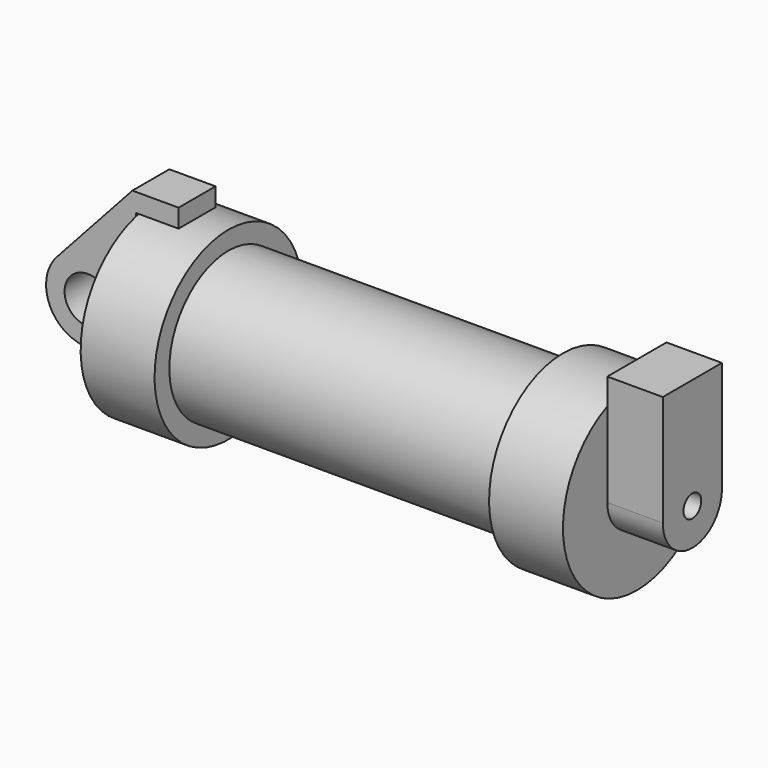
from build123d import *

# Parameters (mm, degrees)
F0_W     = 5.842
F0_H     = 12.7
F0_R     = 3.175
F2_DEPTH = 3.175
F3_R     = 1.524
F4_DEPTH = 7.62


# Not quite as in the source:
# - the program builds the solid bodies; features that only make, move or delete a surface that nothing else refers to are left out


with BuildPart() as f1:
    # F0 (on Front) → F1 (revolve)
    with BuildSketch(Plane.XZ):
        Polygon((5.842, 12.7), (5.842, 0), (66.294, 0), (66.294, 12.7), (56.134, 12.7), (56.134, 10.16), (10.16, 10.16), (10.16, 12.7), align=None)
        with Locations((2.921, 6.35)):
            Rectangle(F0_W, F0_H)
    revolve(axis=Axis((33.147, 0, 0), (-1, 0, 0)))

    # F3 (on face) → F4 (join)
    with BuildSketch(Plane.YZ.offset(66.294)):
        with BuildLine():
            ThreePointArc((-5.08, 0), (0, 5.08), (5.08, 0))
            Line((5.08, 0), (5.08, 11.6397422652))
            ThreePointArc((5.08, 11.6397422652), (0, 12.7), (-5.08, 11.6397422652))
            Line((-5.08, 11.6397422652), (-5.08, 0))
        make_face()
        with BuildLine():
            ThreePointArc((-5.08, 11.6397422652), (0, 12.7), (5.08, 11.6397422652))
            Line((5.08, 11.6397422652), (5.08, 15.24))
            Line((5.08, 15.24), (-5.08, 15.24))
            Line((-5.08, 15.24), (-5.08, 11.6397422652))
        make_face()
        with BuildLine():
            ThreePointArc((-5.08, 0), (0, -5.08), (5.08, 0))
            ThreePointArc((5.08, 0), (0, 5.08), (-5.08, 0))
        make_face()
        Circle(F3_R, mode=Mode.SUBTRACT)
    extrude(amount=F4_DEPTH)


with BuildPart() as f2:
    # F0 (on Front) → F2 (new body, symmetric)
    with BuildSketch(Plane.XZ):
        with BuildLine():
            ThreePointArc((-8.1826630726, -5.5069827884), (-3.1957909266, -4.5493385486), (-0.9398, 0))
            ThreePointArc((-0.9398, 0), (-4.5919612295, 5.3297205562), (-10.8806298187, 3.8475430269))
            ThreePointArc((-10.8806298187, 3.8475430269), (-12.1459778134, -1.5837270034), (-8.1826630726, -5.5069827884))
        make_face()
        with Locations((-6.6548, 0)):
            Circle(F0_R, mode=Mode.SUBTRACT)
        with BuildLine():
            Line((-0.9398, 0), (0, 0))
            Line((0, 0), (0, 12.7))
            Line((0, 12.7), (5.842, 12.7))
            Line((5.842, 12.7), (5.842, 15.24))
            Line((5.842, 15.24), (-0.508, 15.24))
            Line((-0.508, 15.24), (-10.8806298187, 3.8475430269))
            ThreePointArc((-10.8806298187, 3.8475430269), (-4.5919612295, 5.3297205562), (-0.9398, 0))
        make_face()
        with BuildLine():
            Line((5.842, 0), (0, 0))
            Line((0, 0), (-0.9398, 0))
            ThreePointArc((-0.9398, 0), (-3.1957909266, -4.5493385486), (-8.1826630726, -5.5069827884))
            Line((-8.1826630726, -5.5069827884), (5.842, -9.398))
            Line((5.842, -9.398), (5.842, 0))
        make_face()
    extrude(amount=F2_DEPTH, both=True)


solid = Compound([f1.part, f2.part])
